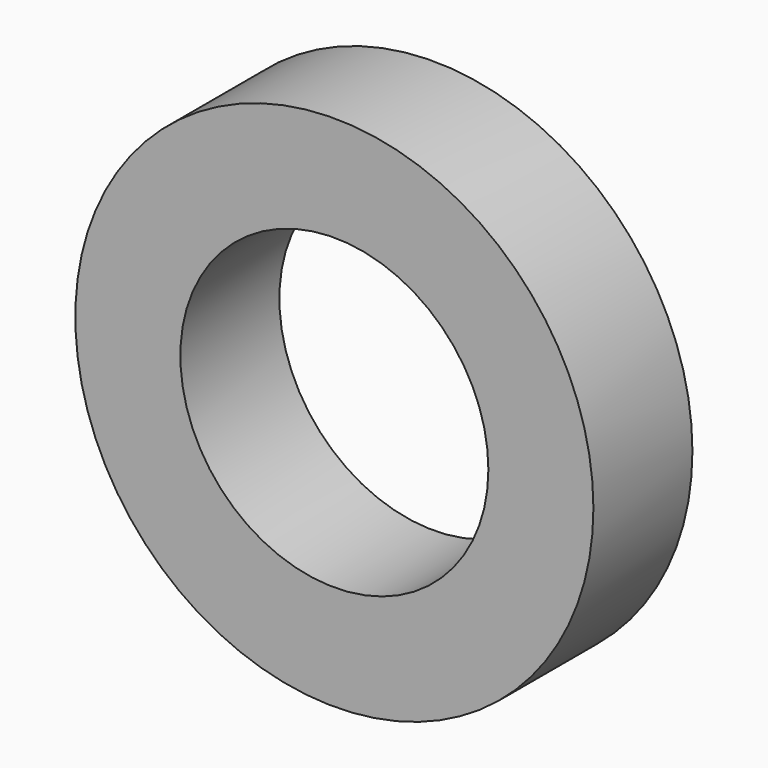
from build123d import *

# Parameters (mm, degrees)
F0_R     = 26.5779703786
F1_DEPTH = 6.35
F4_R     = 15.8016250511
F5_DEPTH = 38.1


# Not quite as in the source:
# - the program builds the solid bodies; features that only make, move or delete a surface that nothing else refers to are left out


with BuildPart() as f1:
    # F0 (on Front) → F1 (new body, symmetric)
    with BuildSketch(Plane.XZ):
        Circle(F0_R)
    extrude(amount=F1_DEPTH, both=True)

    # F4 (on Front) → F5 (cut, symmetric)
    with BuildSketch(Plane.XZ):
        Circle(F4_R)
    extrude(amount=F5_DEPTH, both=True, mode=Mode.SUBTRACT)


solid = f1.part
